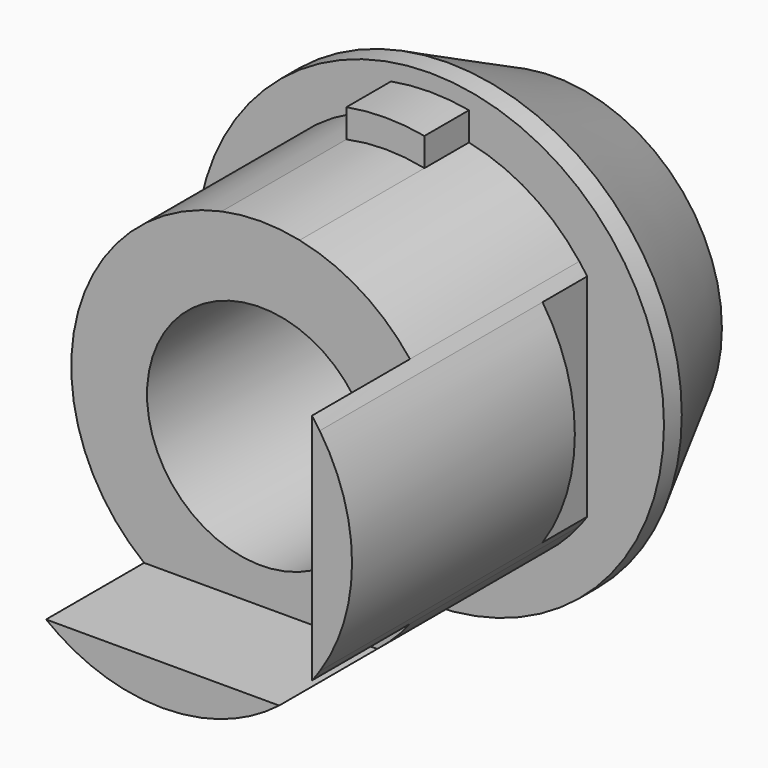
from build123d import *
from build123d import SkipClean  # not in build123d's __all__

# Parameters (mm, degrees)
F0_R     = 10.5
F0_R_2   = 5.1
F1_DEPTH = 7
F2_DEPTH = 2.5
F3_START = 2.5
F3_DEPTH = 7
F4_START = 7
F4_DEPTH = 8
F5_R     = 6.35
F5_R_2   = 5.1
F6_DEPTH = 2.6
F7_SIZE2 = 6
F7_SIZE  = 3


with BuildPart() as f1:
    # F0 (on Front) → F1 (new body)
    with BuildSketch(Plane.XZ):
        Circle(F0_R)
        with BuildLine():
            ThreePointArc((1.75, 9.591663), (7.48749, 6.244998), (9.75, 0))
            ThreePointArc((9.75, 0), (7.48749, -6.244998), (1.75, -9.591663))
            ThreePointArc((1.75, -9.591663), (0, -9.75), (-1.75, -9.591663))
            ThreePointArc((-1.75, -9.591663), (-9.75, 0), (-1.75, 9.591663))
            ThreePointArc((-1.75, 9.591663), (0, 9.75), (1.75, 9.591663))
        make_face(mode=Mode.SUBTRACT)
        with BuildLine():
            Line((-1.75, 8.317902), (-1.75, 9.591663))
            ThreePointArc((-1.75, 9.591663), (-9.75, 0), (-1.75, -9.591663))
            Line((-1.75, -9.591663), (-1.75, -8.317902))
            ThreePointArc((-1.75, -8.317902), (-3.582858, -7.707991), (-5.230679, -6.7))
            ThreePointArc((-5.230679, -6.7), (-6.21739, -5.796039), (-7.05, -4.748421))
            ThreePointArc((-7.05, -4.748421), (-8.5, 0), (-7.05, 4.748421))
            ThreePointArc((-7.05, 4.748421), (-4.748189, 7.050156), (-1.75, 8.317902))
        make_face()
        with BuildLine():
            Line((1.75, 8.317902), (1.75, 9.591663))
            ThreePointArc((1.75, 9.591663), (0, 9.75), (-1.75, 9.591663))
            Line((-1.75, 9.591663), (-1.75, 8.317902))
            ThreePointArc((-1.75, 8.317902), (0, 8.5), (1.75, 8.317902))
        make_face()
        with BuildLine():
            ThreePointArc((1.75, -9.591663), (7.48749, -6.244998), (9.75, 0))
            ThreePointArc((9.75, 0), (7.48749, 6.244998), (1.75, 9.591663))
            Line((1.75, 9.591663), (1.75, 8.317902))
            ThreePointArc((1.75, 8.317902), (4.498151, 7.212256), (6.7, 5.230679))
            ThreePointArc((6.7, 5.230679), (6.879227, 4.992618), (7.05, 4.748421))
            ThreePointArc((7.05, 4.748421), (8.129422, 2.482438), (8.5, 0))
            ThreePointArc((8.5, 0), (8.129422, -2.482438), (7.05, -4.748421))
            ThreePointArc((7.05, -4.748421), (6.879227, -4.992618), (6.7, -5.230679))
            ThreePointArc((6.7, -5.230679), (6.010408, -6.010408), (5.230679, -6.7))
            ThreePointArc((5.230679, -6.7), (3.582858, -7.707991), (1.75, -8.317902))
            Line((1.75, -8.317902), (1.75, -9.591663))
        make_face()
        with BuildLine():
            ThreePointArc((-1.75, -9.591663), (0, -9.75), (1.75, -9.591663))
            Line((1.75, -9.591663), (1.75, -8.317902))
            ThreePointArc((1.75, -8.317902), (0, -8.5), (-1.75, -8.317902))
            Line((-1.75, -8.317902), (-1.75, -9.591663))
        make_face()
        with BuildLine():
            ThreePointArc((-1.75, -8.317902), (0, -8.5), (1.75, -8.317902))
            ThreePointArc((1.75, -8.317902), (3.582858, -7.707991), (5.230679, -6.7))
            Line((5.230679, -6.7), (-5.230679, -6.7))
            ThreePointArc((-5.230679, -6.7), (-3.582858, -7.707991), (-1.75, -8.317902))
        make_face()
        with BuildLine():
            Line((-7.05, -4.748421), (-7.05, 4.748421))
            ThreePointArc((-7.05, 4.748421), (-8.5, 0), (-7.05, -4.748421))
        make_face()
        with BuildLine():
            ThreePointArc((6.7, 5.230679), (4.498151, 7.212256), (1.75, 8.317902))
            ThreePointArc((1.75, 8.317902), (0, 8.5), (-1.75, 8.317902))
            ThreePointArc((-1.75, 8.317902), (-4.748189, 7.050156), (-7.05, 4.748421))
            Line((-7.05, 4.748421), (-7.05, -4.748421))
            ThreePointArc((-7.05, -4.748421), (-6.21739, -5.796039), (-5.230679, -6.7))
            Line((-5.230679, -6.7), (5.230679, -6.7))
            ThreePointArc((5.230679, -6.7), (6.010408, -6.010408), (6.7, -5.230679))
            Line((6.7, -5.230679), (6.7, 5.230679))
        make_face()
        Circle(F0_R_2, mode=Mode.SUBTRACT)
        with BuildLine():
            ThreePointArc((8.5, 0), (8.129422, 2.482438), (7.05, 4.748421))
            Line((7.05, 4.748421), (7.05, -4.748421))
            ThreePointArc((7.05, -4.748421), (8.129422, -2.482438), (8.5, 0))
        make_face()
        with BuildLine():
            ThreePointArc((7.05, 4.748421), (6.879227, 4.992618), (6.7, 5.230679))
            Line((6.7, 5.230679), (6.7, -5.230679))
            ThreePointArc((6.7, -5.230679), (6.879227, -4.992618), (7.05, -4.748421))
            Line((7.05, -4.748421), (7.05, 4.748421))
        make_face()
    extrude(amount=-F1_DEPTH)

    # F0 (on Front) → F2 (join)
    with BuildSketch(Plane.XZ):
        with BuildLine():
            Line((1.75, 8.317902), (1.75, 9.591663))
            ThreePointArc((1.75, 9.591663), (0, 9.75), (-1.75, 9.591663))
            Line((-1.75, 9.591663), (-1.75, 8.317902))
            ThreePointArc((-1.75, 8.317902), (0, 8.5), (1.75, 8.317902))
        make_face()
        with BuildLine():
            ThreePointArc((6.7, 5.230679), (4.498151, 7.212256), (1.75, 8.317902))
            ThreePointArc((1.75, 8.317902), (0, 8.5), (-1.75, 8.317902))
            ThreePointArc((-1.75, 8.317902), (-4.748189, 7.050156), (-7.05, 4.748421))
            Line((-7.05, 4.748421), (-7.05, -4.748421))
            ThreePointArc((-7.05, -4.748421), (-6.21739, -5.796039), (-5.230679, -6.7))
            Line((-5.230679, -6.7), (5.230679, -6.7))
            ThreePointArc((5.230679, -6.7), (6.010408, -6.010408), (6.7, -5.230679))
            Line((6.7, -5.230679), (6.7, 5.230679))
        make_face()
        Circle(F0_R_2, mode=Mode.SUBTRACT)
        with BuildLine():
            ThreePointArc((7.05, 4.748421), (6.879227, 4.992618), (6.7, 5.230679))
            Line((6.7, 5.230679), (6.7, -5.230679))
            ThreePointArc((6.7, -5.230679), (6.879227, -4.992618), (7.05, -4.748421))
            Line((7.05, -4.748421), (7.05, 4.748421))
        make_face()
        with BuildLine():
            ThreePointArc((-1.75, -9.591663), (0, -9.75), (1.75, -9.591663))
            Line((1.75, -9.591663), (1.75, -8.317902))
            ThreePointArc((1.75, -8.317902), (0, -8.5), (-1.75, -8.317902))
            Line((-1.75, -8.317902), (-1.75, -9.591663))
        make_face()
        with BuildLine():
            ThreePointArc((-1.75, -8.317902), (0, -8.5), (1.75, -8.317902))
            ThreePointArc((1.75, -8.317902), (3.582858, -7.707991), (5.230679, -6.7))
            Line((5.230679, -6.7), (-5.230679, -6.7))
            ThreePointArc((-5.230679, -6.7), (-3.582858, -7.707991), (-1.75, -8.317902))
        make_face()
    extrude(amount=F2_DEPTH)

    # F0 (on Front) → F3 (join)
    with BuildSketch(Plane.XZ.offset(F3_START)):
        with BuildLine():
            Line((-7.05, -4.748421), (-7.05, 4.748421))
            ThreePointArc((-7.05, 4.748421), (-8.5, 0), (-7.05, -4.748421))
        make_face()
        with BuildLine():
            ThreePointArc((6.7, 5.230679), (4.498151, 7.212256), (1.75, 8.317902))
            ThreePointArc((1.75, 8.317902), (0, 8.5), (-1.75, 8.317902))
            ThreePointArc((-1.75, 8.317902), (-4.748189, 7.050156), (-7.05, 4.748421))
            Line((-7.05, 4.748421), (-7.05, -4.748421))
            ThreePointArc((-7.05, -4.748421), (-6.21739, -5.796039), (-5.230679, -6.7))
            Line((-5.230679, -6.7), (5.230679, -6.7))
            ThreePointArc((5.230679, -6.7), (6.010408, -6.010408), (6.7, -5.230679))
            Line((6.7, -5.230679), (6.7, 5.230679))
        make_face()
        Circle(F0_R_2, mode=Mode.SUBTRACT)
        with BuildLine():
            ThreePointArc((7.05, 4.748421), (6.879227, 4.992618), (6.7, 5.230679))
            Line((6.7, 5.230679), (6.7, -5.230679))
            ThreePointArc((6.7, -5.230679), (6.879227, -4.992618), (7.05, -4.748421))
            Line((7.05, -4.748421), (7.05, 4.748421))
        make_face()
        with BuildLine():
            ThreePointArc((8.5, 0), (8.129422, 2.482438), (7.05, 4.748421))
            Line((7.05, 4.748421), (7.05, -4.748421))
            ThreePointArc((7.05, -4.748421), (8.129422, -2.482438), (8.5, 0))
        make_face()
        with BuildLine():
            ThreePointArc((-1.75, -8.317902), (0, -8.5), (1.75, -8.317902))
            ThreePointArc((1.75, -8.317902), (3.582858, -7.707991), (5.230679, -6.7))
            Line((5.230679, -6.7), (-5.230679, -6.7))
            ThreePointArc((-5.230679, -6.7), (-3.582858, -7.707991), (-1.75, -8.317902))
        make_face()
    extrude(amount=F3_DEPTH)

    # F0 (on Front) → F4 (join)
    with BuildSketch(Plane.XZ.offset(F4_START)):
        with BuildLine():
            ThreePointArc((-1.75, -8.317902), (0, -8.5), (1.75, -8.317902))
            ThreePointArc((1.75, -8.317902), (3.582858, -7.707991), (5.230679, -6.7))
            Line((5.230679, -6.7), (-5.230679, -6.7))
            ThreePointArc((-5.230679, -6.7), (-3.582858, -7.707991), (-1.75, -8.317902))
        make_face()
        with BuildLine():
            ThreePointArc((7.05, 4.748421), (6.879227, 4.992618), (6.7, 5.230679))
            Line((6.7, 5.230679), (6.7, -5.230679))
            ThreePointArc((6.7, -5.230679), (6.879227, -4.992618), (7.05, -4.748421))
            Line((7.05, -4.748421), (7.05, 4.748421))
        make_face()
        with BuildLine():
            ThreePointArc((8.5, 0), (8.129422, 2.482438), (7.05, 4.748421))
            Line((7.05, 4.748421), (7.05, -4.748421))
            ThreePointArc((7.05, -4.748421), (8.129422, -2.482438), (8.5, 0))
        make_face()
    with SkipClean():  # cleaning this boolean's faces spoils the solid; the shape is the same uncleaned
        extrude(amount=F4_DEPTH)

    # F5 (on face) → F6 (cut)
    with BuildSketch(Plane(origin=(0, 7, 0), x_dir=(-1, 0, 0), z_dir=(0, 1, 0))):
        Circle(F5_R)
        Circle(F5_R_2, mode=Mode.SUBTRACT)
    with SkipClean():  # cleaning this boolean's faces spoils the solid; the shape is the same uncleaned
        extrude(amount=-F6_DEPTH, mode=Mode.SUBTRACT)

    # F7
    f7_edges = [f1.edges().sort_by_distance(p)[0] for p in [
        (-10.5, 7, 0),
    ]]
    f7_side = f1.faces().sort_by_distance((-10.203015, 7, 0))[0]
    chamfer(f7_edges, length=F7_SIZE, length2=F7_SIZE2, reference=f7_side)


solid = f1.part
